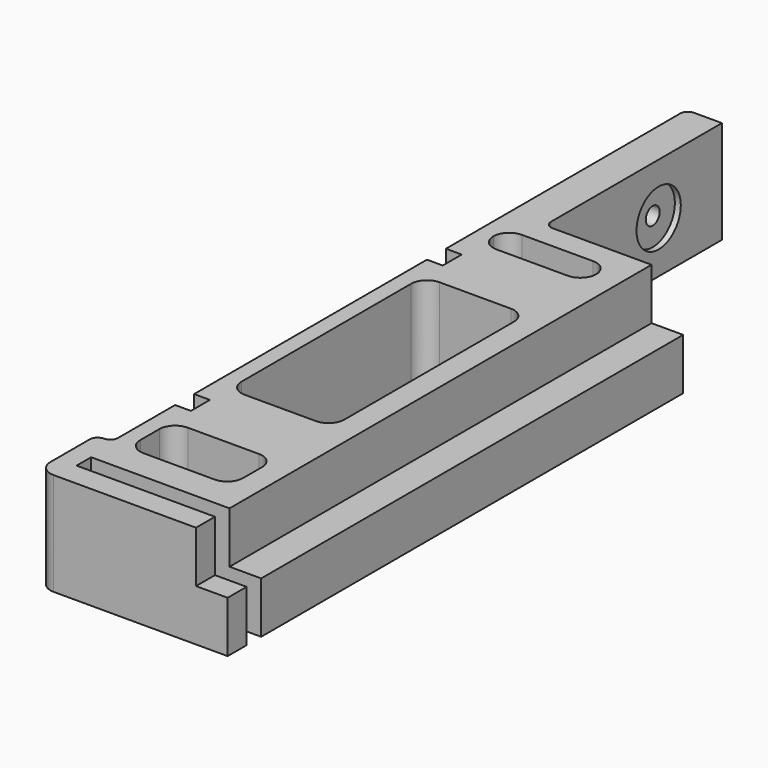
from build123d import *

# Parameters (mm, degrees)
F0_W      = 13
F0_H      = 7
F0_H_2    = 30.8050829545
F0_H_3    = 4
F1_DEPTH  = 13
F3_R      = 1.99999
F4_R      = 0.99999
F5_D      = 2.2
F7_W      = 3
F7_H      = 6.5
F6_W      = 66.7
F6_H      = 6.5
F8_DEPTH  = 2
F9_DEPTH  = 2
F10_R     = 3.5
F10_R_2   = 1.1
F11_DEPTH = 0.75


# Not quite as in the source:
# - a fillet or chamfer is up to 0.001 mm smaller than in the source, because OpenCascade refuses the exact size


with BuildPart() as f1:
    # F0 (on Top) → F1 (new body)
    with BuildSketch(Plane.XY):
        Polygon((-22, 0), (0, 0), (0, 3), (-19.5, 3), (-19.5, 5.3), (0, 5.3), (0, 72), (-15.5, 72), (-15.5, 100), (-20, 100), (-20, 62), (-18, 62), (-18, 59), (-20, 59), (-20, 22.1949170455), (-18, 22.1949170455), (-18, 19.1949170455), (-20, 19.1949170455), (-20, 9.1949170455), (-22, 9.1949170455), align=None)
        with Locations((-11.5, 12.6949170455)):
            Rectangle(F0_W, F0_H, mode=Mode.SUBTRACT)
        with Locations((-11.5, 40.5974585228)):
            Rectangle(F0_W, F0_H_2, mode=Mode.SUBTRACT)
        with Locations((-11.5, 67)):
            Rectangle(F0_W, F0_H_3, mode=Mode.SUBTRACT)
    extrude(amount=F1_DEPTH)

    # F3 (radius 2 in the source; OpenCascade refuses exactly that, so slightly less here)
    f3_edges = [f1.edges().sort_by_distance(p)[0] for p in [
        (-22, 0, 6.5),
        (-18, 69, 6.5),
        (-18, 65, 6.5),
        (-5, 69, 6.5),
        (-5, 65, 6.5),
        (-18, 56, 6.5),
        (-5, 56, 6.5),
        (-18, 25.194917, 6.5),
        (-5, 25.194917, 6.5),
        (-18, 9.194917, 6.5),
        (-5, 9.194917, 6.5),
        (-5, 16.194917, 6.5),
        (-18, 16.194917, 6.5),
    ]]
    fillet(f3_edges, radius=F3_R)

    # F4 (radius 1 in the source; OpenCascade refuses exactly that, so slightly less here)
    f4_edges = [f1.edges().sort_by_distance(p)[0] for p in [
        (-15.5, 72, 6.5),
        (-20, 100, 6.5),
        (-22, 9.194917, 6.5),
        (-20, 9.194917, 6.5),
    ]]
    fillet(f4_edges, radius=F4_R)

    # F5 (through all)
    with Locations(Plane(origin=(-20, 0, 0), x_dir=(0, -1, 0), z_dir=(-1, 0, 0))):
        with Locations((-90, 6.5)):
            Hole(F5_D / 2)

    # F7 (on face) + F6 (on face) → F8 (join)
    with BuildSketch(Plane.YZ):
        with Locations((1.5, 3.25)):
            Rectangle(F7_W, F7_H)
    with BuildSketch(Plane.YZ):
        with Locations((38.65, 3.25)):
            Rectangle(F6_W, F6_H)
    extrude(amount=F8_DEPTH)

    # F9 (cut): faces of the model
    f9_faces = [f1.faces().sort_by_distance(p)[0] for p in [
        (0, 1.5, 9.75),
        (0, 38.65, 9.75),
    ]]
    extrude(f9_faces, amount=-F9_DEPTH, mode=Mode.SUBTRACT)

    # F10 (on face) → F11 (cut)
    with BuildSketch(Plane.YZ.offset(-15.5)):
        with Locations((90, 6.5)):
            Circle(F10_R)
        with Locations((90, 6.5)):
            Circle(F10_R_2, mode=Mode.SUBTRACT)
    extrude(amount=-F11_DEPTH, mode=Mode.SUBTRACT)


solid = f1.part
